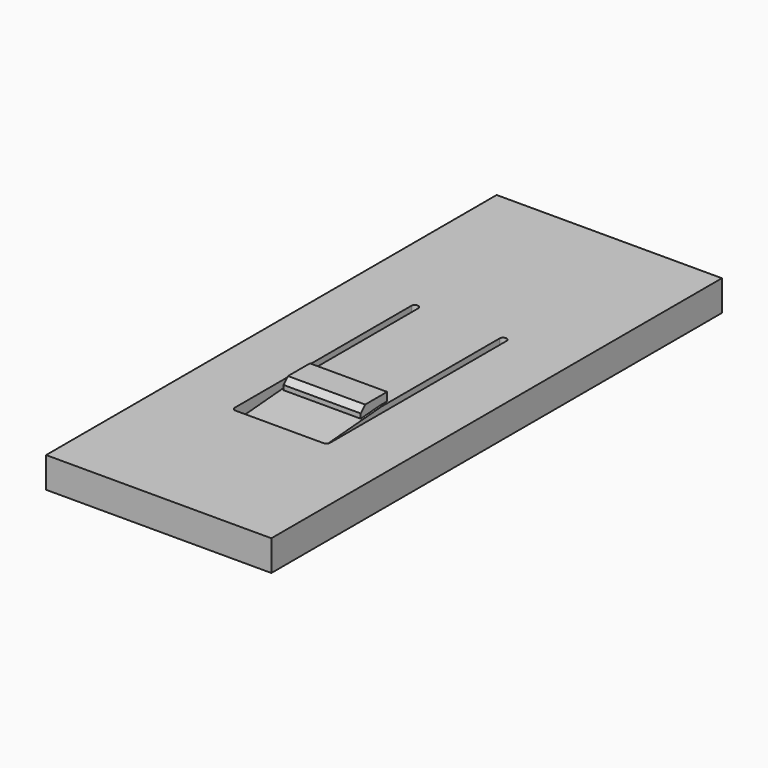
from build123d import *

# Parameters (mm, degrees)
F0_W         = 16.2
F0_H         = 40.5
F1_DEPTH     = 2.2
F0_W_2       = 5.85
F0_H_2       = 15.625
F0_W_3       = 5.55
F0_H_3       = 2.375
F2_DEPTH     = 1.8
F3_DEPTH     = 0.6
F4_T1_DEPTH  = 5.85
F4_T6_DEPTH  = 18.8484687937
F4_T11_DEPTH = 5.85
F4_T16_DEPTH = 18.8484687937
F5_SIZE      = 0.39999


# Not quite as in the source:
# - a fillet or chamfer that OpenCascade refuses, or shapes differently, is made with other operations: its cross-section is extruded or revolved along the edge and cut away or added
# - a fillet or chamfer is up to 0.001 mm smaller than in the source, because OpenCascade refuses the exact size


with BuildPart() as f1:
    # F0 (on Top) → F1 (new body)
    with BuildSketch(Plane.XY):
        with Locations((8.1, 20.25)):
            Rectangle(F0_W, F0_H)
        with BuildLine():
            Line((11.275, 10.8625), (4.925, 10.8625))
            ThreePointArc((4.925, 10.8625), (4.7482233047, 10.9357233047), (4.675, 11.1125))
            Line((4.675, 11.1125), (4.675, 26.9875))
            ThreePointArc((4.675, 26.9875), (4.925, 27.2375), (5.175, 26.9875))
            Line((5.175, 26.9875), (11.025, 26.9875))
            ThreePointArc((11.025, 26.9875), (11.275, 27.2375), (11.525, 26.9875))
            Line((11.525, 26.9875), (11.525, 11.1125))
            ThreePointArc((11.525, 11.1125), (11.4517766953, 10.9357233047), (11.275, 10.8625))
        make_face(mode=Mode.SUBTRACT)
    extrude(amount=-F1_DEPTH)

    # F0 (on Top) → F2 (join)
    with BuildSketch(Plane.XY):
        with Locations((8.1, 19.175)):
            Rectangle(F0_W_2, F0_H_2)
        with Locations((8.1, 15.875)):
            Rectangle(F0_W_3, F0_H_3, mode=Mode.SUBTRACT)
        with Locations((8.1, 15.875)):
            Rectangle(F0_W_3, F0_H_3)
    extrude(amount=-F2_DEPTH)

    # F0 (on Top) → F3 (join)
    with BuildSketch(Plane.XY):
        with Locations((8.1, 15.875)):
            Rectangle(F0_W_3, F0_H_3)
    extrude(amount=F3_DEPTH)

    # F4: chamfer of 5 x 0.4 on 2 edges, made by hand

    # F4_s2 → F4_t1 (cut)
    with BuildSketch(Plane.YZ.offset(5.175)):
        Polygon((11.3625, -1.4), (16.3625, -1.8), (11.3625, -1.8), align=None)
    extrude(amount=F4_T1_DEPTH, mode=Mode.SUBTRACT)


with BuildPart() as f4_tool4:
    # F4_s5 → F4_t6 (new body)
    with BuildSketch(Plane.YZ.offset(5.175)):
        Polygon((16.3625, 0), (11.3625, -0.4), (11.3625, 0), align=None)
    extrude(amount=F4_T6_DEPTH)

    split(bisect_by=Plane.YZ.offset(5.325), keep=Keep.BOTTOM)


with BuildPart() as f1_1:
    add(f1.part)

    # F4_t3: cut F4_tool4
    add(f4_tool4.part, mode=Mode.SUBTRACT)


with BuildPart() as f4_tool9:
    # F4_s10 → F4_t11 (new body)
    with BuildSketch(Plane.YZ.offset(5.175)):
        Polygon((16.3625, 0), (11.3625, -0.4), (11.3625, 0), align=None)
    extrude(amount=F4_T11_DEPTH)

    split(bisect_by=Plane.XZ.offset(-14.6875), keep=Keep.TOP)


with BuildPart() as f1_2:
    add(f1_1.part)

    # F4_t8: cut F4_tool9
    add(f4_tool9.part, mode=Mode.SUBTRACT)


with BuildPart() as f4_tool14:
    # F4_s15 → F4_t16 (new body)
    with BuildSketch(Plane.YZ.offset(-7.8234687937)):
        Polygon((16.3625, 0), (11.3625, -0.4), (11.3625, 0), align=None)
    extrude(amount=F4_T16_DEPTH)

    split(bisect_by=Plane.YZ.offset(10.875), keep=Keep.TOP)


with BuildPart() as f1_3:
    add(f1_2.part)

    # F4_t13: cut F4_tool14
    add(f4_tool14.part, mode=Mode.SUBTRACT)

    # F5 (size 0.4 in the source; OpenCascade refuses exactly that, so slightly less here)
    f5_edges = [f1_3.edges().sort_by_distance(p)[0] for p in [
        (8.1, 14.6875, 0.6),
        (8.1, 26.9875, -1.8),
    ]]
    chamfer(f5_edges, length=F5_SIZE)


solid = f1_3.part
